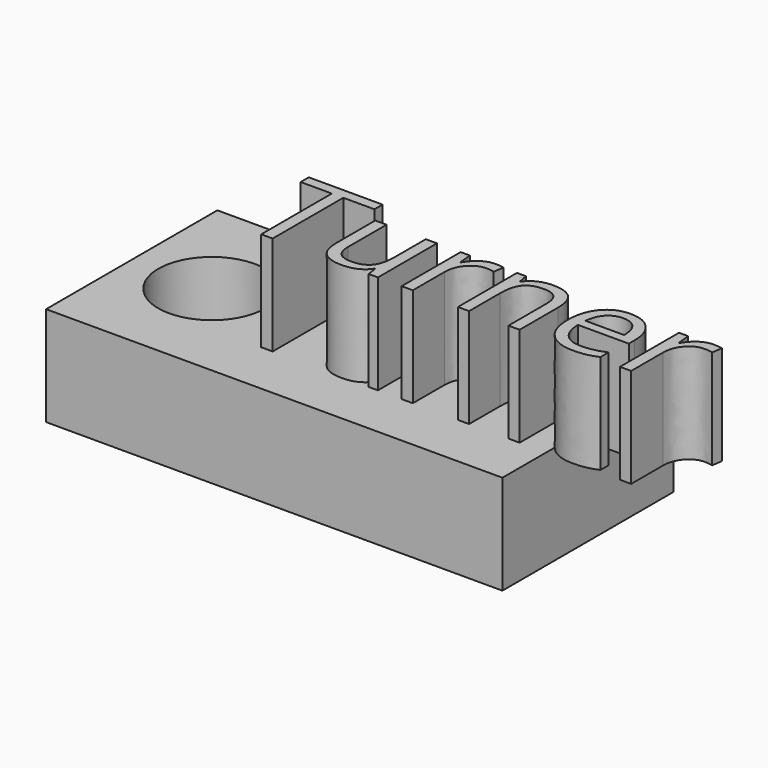
from build123d import *

# Parameters (mm, degrees)
F0_W         = 116.5613345802
F0_H         = 54.6830911189
F1_DEPTH     = 25.4
F2_R         = 13.6780945515
F3_DEPTH     = 25.4
F4_TEXT_SIZE = 35.2262959091
F5_DEPTH     = 25.4


# Not quite as in the source:
# - Text() gives the source's letters only with a copy of the font that has no kerning and outlines rounded to 1/6400 em; it was checked with that copy


with BuildPart() as f1:
    # F0 (on Top) → F1 (new body)
    with BuildSketch(Plane.XY):
        with Locations((0.2878066152, 13.3829666302)):
            Rectangle(F0_W, F0_H)
    extrude(amount=F1_DEPTH)

    # F2 (on face) → F3 (cut)
    with BuildSketch(Plane.XY.offset(25.4)):
        with Locations((-37.7324670553, 13.6385764927)):
            Circle(F2_R)
    extrude(amount=-F3_DEPTH, mode=Mode.SUBTRACT)

    # F4 (on face) → F5 (join)
    with BuildSketch(Plane.XY.offset(25.4)):
        with Locations((-22.4794540554, 0)):
            Text('Turner', F4_TEXT_SIZE, font='Open Sans', text_align=(TextAlign.LEFT, TextAlign.BOTTOM))
    extrude(amount=F5_DEPTH)


solid = f1.part
